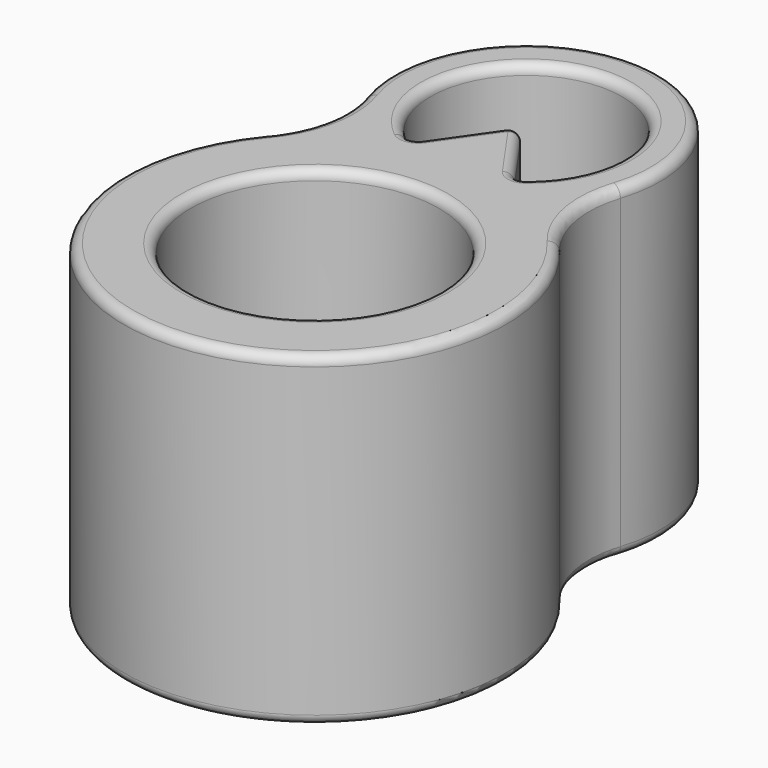
from build123d import *

# Parameters (mm, degrees)
F0_R     = 6.475
F1_DEPTH = 17
F2_R     = 5.5
F3_R     = 0.5


with BuildPart() as f1:
    # F0 (on Top) → F1 (new body)
    with BuildSketch(Plane.XY):
        with BuildLine():
            ThreePointArc((4.8262190603, 8.7297327899), (0, 20.8), (-4.8262190603, 8.7297327899))
            ThreePointArc((-4.8262190603, 8.7297327899), (0, -9.975), (4.8262190603, 8.7297327899))
        make_face()
        Circle(F0_R, mode=Mode.SUBTRACT)
        with BuildLine():
            ThreePointArc((-3.1450929018, 9.9130486704), (0, 18.8), (3.1450929018, 9.9130486704))
            ThreePointArc((3.1450929018, 9.9130486704), (2.7608172994, 9.8066350661), (2.4209107257, 10.0150939708))
            Line((2.4209107257, 10.0150939708), (0.409672886, 12.8895055936))
            ThreePointArc((0.409672886, 12.8895055936), (0, 13.1028557611), (-0.409672886, 12.8895055936))
            Line((-0.409672886, 12.8895055936), (-2.4209107257, 10.0150939708))
            ThreePointArc((-2.4209107257, 10.0150939708), (-2.7608172994, 9.8066350661), (-3.1450929018, 9.9130486704))
        make_face(mode=Mode.SUBTRACT)
    extrude(amount=F1_DEPTH)

    # F2
    f2_edges = [f1.edges().sort_by_distance(p)[0] for p in [
        (-4.826219, 8.729733, 8.5),
        (4.826219, 8.729733, 8.5),
    ]]
    fillet(f2_edges, radius=F2_R)

    # F3
    f3_edges = [f1.edges().sort_by_distance(p)[0] for p in [
        (0, 18.8, 17),
        (-1.415292, 11.4523, 17),
        (-2.760817, 9.806635, 17),
        (1.415292, 11.4523, 17),
        (0, 13.102856, 17),
        (2.760817, 9.806635, 17),
        (6.479776, 8.878156, 17),
        (0, 20.8, 17),
        (-6.475, 0, 17),
        (-6.475, 0, 0),
        (0, 18.8, 0),
        (0, -9.975, 0),
        (0, -9.975, 17),
        (-6.479776, 8.878156, 0),
        (6.479776, 8.878156, 0),
        (0, 20.8, 0),
        (-2.760817, 9.806635, 0),
        (2.760817, 9.806635, 0),
        (1.415292, 11.4523, 0),
        (0, 13.102856, 0),
        (-1.415292, 11.4523, 0),
        (-6.479776, 8.878156, 17),
    ]]
    fillet(f3_edges, radius=F3_R)


solid = f1.part
